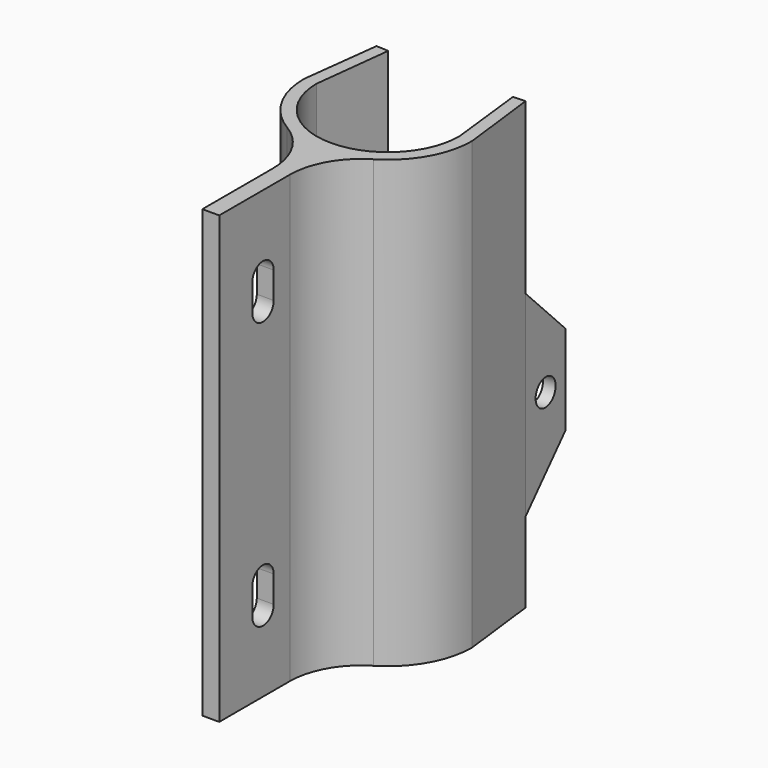
from build123d import *

# Parameters (mm, degrees)
F1_DEPTH  = 1.5
F2_DEPTH  = 50
F3_R      = 8
F4_W      = 1.3695214008
F4_H      = 10
F6_DEPTH  = 6
F5_W      = 1.3695214008
F5_H      = 10
F7_DEPTH  = 6
F8_R      = 1.5
F9_DEPTH  = 2
F10_R     = 1.5
F11_DEPTH = 2
F12_SIZE  = 5.99999
F14_DEPTH = 3


# Not quite as in the source:
# - a fillet or chamfer is up to 0.001 mm smaller than in the source, because OpenCascade refuses the exact size


with BuildPart() as f1:
    # F0 (on Top) → F1 (new body)
    with BuildSketch(Plane.XY):
        with BuildLine():
            Line((-8.8714406544, -8.0876392549), (-13.1571549401, -8.0876392549))
            ThreePointArc((-13.1571549401, -8.0876392549), (-5.1571549401, -16.0876392549), (2.8428450599, -8.0876392549))
            Line((2.8428450599, -8.0876392549), (-1.4428692258, -8.0876392549))
            Line((-1.4428692258, -8.0876392549), (-8.8714406544, -8.0876392549))
        make_face()
    extrude(amount=F1_DEPTH)

    # F0 (on Top) → F2 (join)
    with BuildSketch(Plane.XY):
        with BuildLine():
            ThreePointArc((2.8428450599, -8.0876392549), (-5.1571549401, -16.0876392549), (-13.1571549401, -8.0876392549))
            Line((-13.1571549401, -8.0876392549), (-12.1455313702, 0.680061955))
            Line((-12.1455313702, 0.680061955), (-13.5133440803, 0.7484524309))
            Line((-13.5133440803, 0.7484524309), (-14.5857263686, -8.0876392549))
            ThreePointArc((-14.5857263686, -8.0876392549), (-12.1513540266, -14.4105450997), (-6.1053030882, -17.4684161029))
            Line((-6.1053030882, -17.4684161029), (-6.1053030882, -32.9236180908))
            Line((-6.1053030882, -32.9236180908), (-4.2090067919, -32.9236180908))
            Line((-4.2090067919, -32.9236180908), (-4.2090067919, -17.4684161029))
            ThreePointArc((-4.2090067919, -17.4684161029), (1.8370441464, -14.4105450997), (4.2714164885, -8.0876392549))
            Line((4.2714164885, -8.0876392549), (3.1990342002, 0.7484524309))
            Line((3.1990342002, 0.7484524309), (1.83122149, 0.680061955))
            Line((1.83122149, 0.680061955), (2.8428450599, -8.0876392549))
        make_face()
    extrude(amount=F2_DEPTH)

    # F3
    f3_edges = [f1.edges().sort_by_distance(p)[0] for p in [
        (-6.105303, -17.468416, 25),
        (-4.209007, -17.468416, 25),
    ]]
    fillet(f3_edges, radius=F3_R)

    # F4 (on face) → F6 (join)
    with BuildSketch(Plane(origin=(-0.0293516073, 0.5870335173, 0), x_dir=(-0.9987523447, -0.0499375007, 0), z_dir=(-0.0499375007, 0.9987523447, 0))):
        with Locations((-2.5476580515, 20)):
            Rectangle(F4_W, F4_H)
    extrude(amount=F6_DEPTH)

    # F5 (on face) → F7 (join)
    with BuildSketch(Plane(origin=(0.0036302561, 0.0726052918, 0), x_dir=(-0.9987523447, 0.0499375007, 0), z_dir=(0.0499375007, 0.9987523447, 0))):
        with Locations((12.8490992282, 20)):
            Rectangle(F5_W, F5_H)
    extrude(amount=F7_DEPTH)

    # F8 (on face) → F9 (cut)
    with BuildSketch(Plane(origin=(3.2283858075, 0.1614189135, 0), x_dir=(-0.0499375007, 0.9987523447, 0), z_dir=(0.9987523447, 0.0499375007, 0))):
        with Locations((3.5877668478, 20)):
            Circle(F8_R)
    extrude(amount=-F9_DEPTH, mode=Mode.SUBTRACT)

    # F10 (on face) → F11 (cut)
    with BuildSketch(Plane(origin=(-13.5169743364, 0.6758471391, 0), x_dir=(-0.0499375007, -0.9987523447, 0), z_dir=(-0.9987523447, 0.0499375007, 0))):
        with Locations((-3.0726959913, 20)):
            Circle(F10_R)
    extrude(amount=-F11_DEPTH, mode=Mode.SUBTRACT)

    # F12 (size 6 in the source; OpenCascade refuses exactly that, so slightly less here)
    f12_edges = [f1.edges().sort_by_distance(p)[0] for p in [
        (2.515128, 0.714257, 15),
        (-12.829438, 0.714257, 15),
        (2.515128, 0.714257, 25),
        (-12.829438, 0.714257, 25),
    ]]
    chamfer(f12_edges, length=F12_SIZE)

    # F13 (on face) → F14 (cut)
    with BuildSketch(Plane.YZ.offset(-4.2090067919)):
        with BuildLine():
            ThreePointArc((-28.2929875813, 38.5), (-26.7929875813, 37), (-25.2929875813, 38.5))
            Line((-25.2929875813, 38.5), (-25.2929875813, 41.5))
            ThreePointArc((-25.2929875813, 41.5), (-26.7929875813, 43), (-28.2929875813, 41.5))
            Line((-28.2929875813, 41.5), (-28.2929875813, 38.5))
        make_face()
        with BuildLine():
            ThreePointArc((-28.2929875813, 8.5), (-26.7929875813, 7), (-25.2929875813, 8.5))
            Line((-25.2929875813, 8.5), (-25.2929875813, 11.5))
            ThreePointArc((-25.2929875813, 11.5), (-26.7929875813, 13), (-28.2929875813, 11.5))
            Line((-28.2929875813, 11.5), (-28.2929875813, 8.5))
        make_face()
    extrude(amount=-F14_DEPTH, mode=Mode.SUBTRACT)


solid = f1.part
